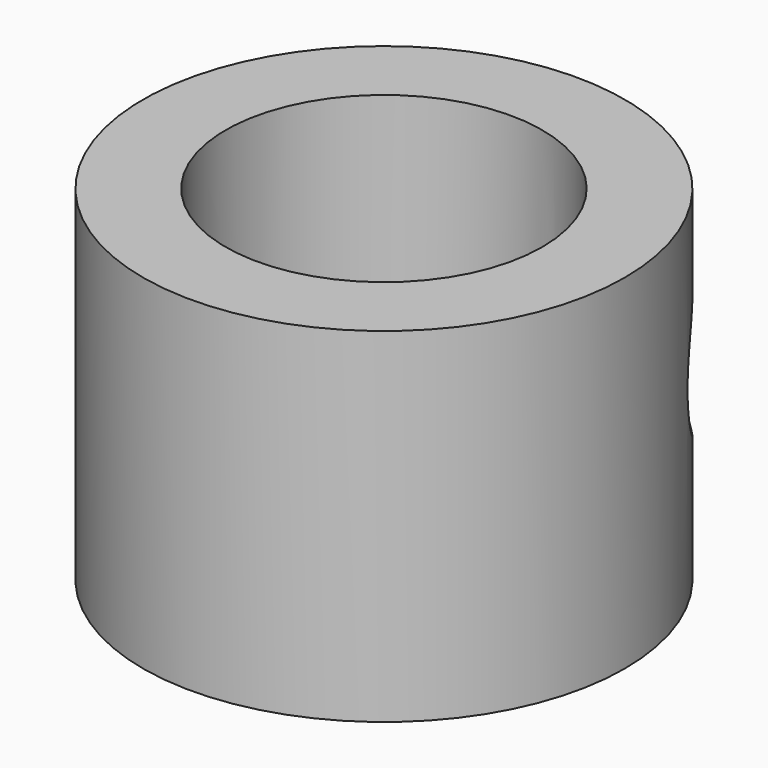
from build123d import *

# Parameters (mm, degrees)
F0_R     = 17.78
F0_R_2   = 11.684
F1_DEPTH = 25.4
F6_R     = 5.08
F7_DEPTH = 12.7


with BuildPart() as f1:
    # F0 (on Top) → F1 (new body)
    with BuildSketch(Plane.XY):
        Circle(F0_R)
        Circle(F0_R_2, mode=Mode.SUBTRACT)
    extrude(amount=F1_DEPTH)

    # F6 (on face) → F7 (cut, symmetric)
    with BuildSketch(Plane(origin=(12.4821024484, 12.4821024484, 0), x_dir=(0.7071067812, -0.7071067812, 0), z_dir=(-0.7071067812, -0.7071067812, 0))):
        with Locations((0, 13.97)):
            Circle(F6_R)
    extrude(amount=F7_DEPTH, both=True, mode=Mode.SUBTRACT)


solid = f1.part
